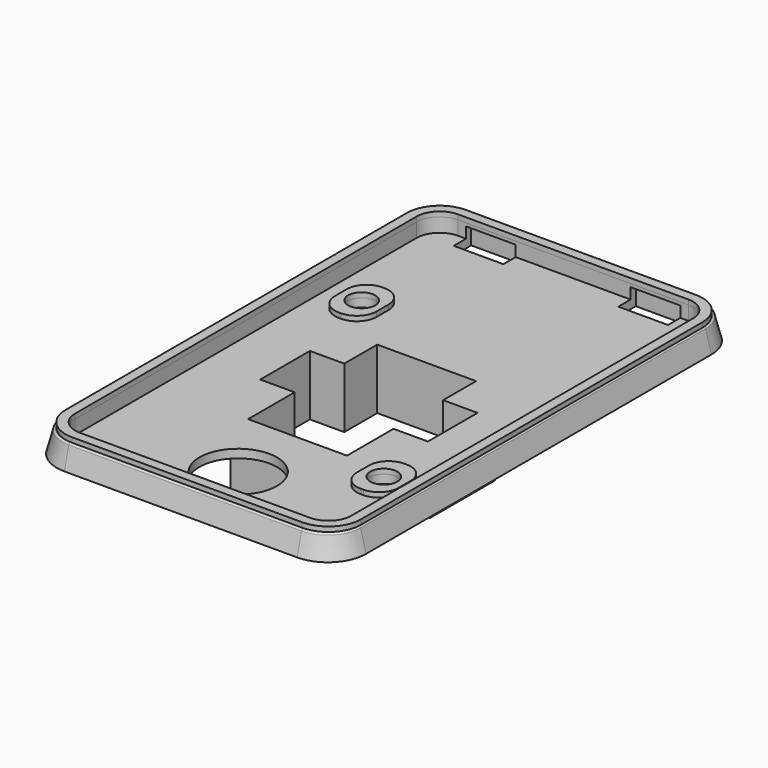
from build123d import *

# Parameters (mm, degrees)
F1_DEPTH     = 1
F4_DEPTH     = 4.64
F5_T1_DEPTH  = 48
F5_T3_DEPTH  = 89
F5_T6_ANGLE  = 90
F5_T8_ANGLE  = 90
F5_T10_ANGLE = 90
F5_T12_ANGLE = 90
F7_DEPTH     = 2.89
F8_R         = 0.4
F9_W         = 10.25
F9_H         = 4.5
F9_R         = 8
F9_R_2       = 2.8
F10_DEPTH    = 4
F11_R        = 2.7984324094
F11_R_2      = 2.7977753944
F12_DEPTH    = 1
F14_DEPTH    = 12.44
F16_DEPTH    = 1.75


# Not quite as in the source:
# - a fillet or chamfer that OpenCascade refuses, or shapes differently, is made with other operations: its cross-section is extruded or revolved along the edge and cut away or added


with BuildPart() as f1:
    # F0 (on Top) → F1 (new body)
    with BuildSketch(Plane.XY):
        with BuildLine():
            Line((23.75, 50.78), (0, 50.78))
            Line((0, 50.78), (-23.75, 50.78))
            ThreePointArc((-23.75, 50.78), (-28.522970773, 48.802970773), (-30.5, 44.03))
            Line((-30.5, 44.03), (-30.5, -44.03))
            ThreePointArc((-30.5, -44.03), (-28.522970773, -48.802970773), (-23.75, -50.78))
            Line((-23.75, -50.78), (0, -50.78))
            Line((0, -50.78), (23.75, -50.78))
            ThreePointArc((23.75, -50.78), (28.522970773, -48.802970773), (30.5, -44.03))
            Line((30.5, -44.03), (30.5, 44.03))
            ThreePointArc((30.5, 44.03), (28.522970773, 48.802970773), (23.75, 50.78))
        make_face()
        with BuildLine():
            Line((-23.75, 48.78), (0, 48.78))
            Line((0, 48.78), (23.75, 48.78))
            ThreePointArc((23.75, 48.78), (27.1087572106, 47.3887572106), (28.5, 44.03))
            Line((28.5, 44.03), (28.5, -44.03))
            ThreePointArc((28.5, -44.03), (27.1087572106, -47.3887572106), (23.75, -48.78))
            Line((23.75, -48.78), (0, -48.78))
            Line((0, -48.78), (-23.75, -48.78))
            ThreePointArc((-23.75, -48.78), (-27.1087572106, -47.3887572106), (-28.5, -44.03))
            Line((-28.5, -44.03), (-28.5, 44.03))
            ThreePointArc((-28.5, 44.03), (-27.1087572106, 47.3887572106), (-23.75, 48.78))
        make_face(mode=Mode.SUBTRACT)
    extrude(amount=F1_DEPTH)


with BuildPart() as f4:
    # F3 (on offset) → F4 (new body, through all)
    with BuildSketch(Plane(origin=(0, 0, -4.64), x_dir=(1, 0, 0), z_dir=(0, 0, -1))):
        with BuildLine():
            Line((24, 52.5), (0, 52.5))
            Line((0, 52.5), (-24, 52.5))
            ThreePointArc((-24, 52.5), (-29.6568542495, 50.1568542495), (-32, 44.5))
            Line((-32, 44.5), (-32, 0))
            Line((-32, 0), (-32, -44.5))
            ThreePointArc((-32, -44.5), (-29.6568542495, -50.1568542495), (-24, -52.5))
            Line((-24, -52.5), (0, -52.5))
            Line((0, -52.5), (24, -52.5))
            ThreePointArc((24, -52.5), (29.6568542495, -50.1568542495), (32, -44.5))
            Line((32, -44.5), (32, 0))
            Line((32, 0), (32, 44.5))
            ThreePointArc((32, 44.5), (29.6568542495, 50.1568542495), (24, 52.5))
        make_face()
    extrude(amount=-F4_DEPTH)

    # F5: chamfer of 1.3 x 5 on 8 edges, made by hand

    # F5_s2 → F5_t1 (cut)
    with BuildSketch(Plane.YZ.offset(-24)):
        Polygon((51.2, 0), (52.5, -5), (52.5, 0), align=None)
        Polygon((-51.2, 0), (-52.5, -5), (-52.5, 0), align=None)
    extrude(amount=F5_T1_DEPTH, mode=Mode.SUBTRACT)

    # F5_s4 → F5_t3 (cut)
    with BuildSketch(Plane.XZ.offset(-44.5)):
        Polygon((-30.7, 0), (-32, -5), (-32, 0), align=None)
        Polygon((30.7, 0), (32, -5), (32, 0), align=None)
    extrude(amount=F5_T3_DEPTH, mode=Mode.SUBTRACT)

    # F5_s5 → F5_t6 (revolve, cut)
    with BuildSketch(Plane.XZ.offset(44.5)):
        Polygon((32, -5), (30.7, 0), (32, 0), align=None)
    revolve(axis=Axis((24, -44.5, 0), (0, 0, -1)), revolution_arc=F5_T6_ANGLE, mode=Mode.SUBTRACT)

    # F5_s7 → F5_t8 (revolve, cut)
    with BuildSketch(Plane.YZ.offset(-24)):
        Polygon((-51.2, 0), (-52.5, -5), (-52.5, 0), align=None)
    revolve(axis=Axis((-24, -44.5, 0), (0, 0, -1)), revolution_arc=F5_T8_ANGLE, mode=Mode.SUBTRACT)

    # F5_s9 → F5_t10 (revolve, cut)
    with BuildSketch(Plane.XZ.offset(-44.5)):
        Polygon((-30.7, 0), (-32, -5), (-32, 0), align=None)
    revolve(axis=Axis((-24, 44.5, 0), (0, 0, -1)), revolution_arc=F5_T10_ANGLE, mode=Mode.SUBTRACT)

    # F5_s11 → F5_t12 (revolve, cut)
    with BuildSketch(Plane.YZ.offset(24)):
        Polygon((51.2, 0), (52.5, -5), (52.5, 0), align=None)
    revolve(axis=Axis((24, 44.5, 0), (0, 0, -1)), revolution_arc=F5_T12_ANGLE, mode=Mode.SUBTRACT)

    # F6 (on Top) → F7 (cut)
    with BuildSketch(Plane.XY):
        with BuildLine():
            Line((23.75, 48.78), (0, 48.78))
            Line((0, 48.78), (-23.75, 48.78))
            ThreePointArc((-23.75, 48.78), (-27.1087572106, 47.3887572106), (-28.5, 44.03))
            Line((-28.5, 44.03), (-28.5, -44.03))
            ThreePointArc((-28.5, -44.03), (-27.1087572106, -47.3887572106), (-23.75, -48.78))
            Line((-23.75, -48.78), (0, -48.78))
            Line((0, -48.78), (23.75, -48.78))
            ThreePointArc((23.75, -48.78), (27.1087572106, -47.3887572106), (28.5, -44.03))
            Line((28.5, -44.03), (28.5, 44.03))
            ThreePointArc((28.5, 44.03), (27.1087572106, 47.3887572106), (23.75, 48.78))
        make_face()
    extrude(amount=-F7_DEPTH, mode=Mode.SUBTRACT)

    # F8
    f8_edges = [f4.edges().sort_by_distance(p)[0] for p in [
        (0, -51.2, 0),
        (30.7, 0, 0),
        (28.737615, 49.237615, 0),
        (28.737615, -49.237615, 0),
        (0, 51.2, 0),
        (-28.737615, 49.237615, 0),
        (-30.7, 0, 0),
        (-28.737615, -49.237615, 0),
    ]]
    fillet(f8_edges, radius=F8_R)

    # F9 (on face) → F10 (cut)
    with BuildSketch(Plane(origin=(0, 0, -4.64), x_dir=(1, 0, 0), z_dir=(0, 0, -1))):
        with Locations((-16.9814, 47.8564)):
            Rectangle(F9_W, F9_H)
        with Locations((16.9814, 47.8564)):
            Rectangle(F9_W, F9_H)
        with Locations((-16.9814, -47.8564)):
            Rectangle(F9_W, F9_H)
        with Locations((16.9814, -47.8564)):
            Rectangle(F9_W, F9_H)
        with Locations((0, 37.5964)):
            Circle(F9_R)
        with Locations((20.6064, 25.8064)):
            Circle(F9_R_2)
        with Locations((-20.6064, -20.0064)):
            Circle(F9_R_2)
    extrude(amount=-F10_DEPTH, mode=Mode.SUBTRACT)

    # F11 (on face) → F12 (join)
    with BuildSketch(Plane.XY.offset(-2.89)):
        with BuildLine():
            Line((20.8564, -20.2064), (20.3564, -20.2064))
            ThreePointArc((20.3564, -20.2064), (17.4926175362, -21.3926175362), (16.3064, -24.2564))
            Line((16.3064, -24.2564), (16.3064, -27.3564))
            ThreePointArc((16.3064, -27.3564), (17.4926175362, -30.2201824638), (20.3564, -31.4064))
            Line((20.3564, -31.4064), (20.8564, -31.4064))
            ThreePointArc((20.8564, -31.4064), (23.7201824638, -30.2201824638), (24.9064, -27.3564))
            Line((24.9064, -27.3564), (24.9064, -24.2564))
            ThreePointArc((24.9064, -24.2564), (23.7201824638, -21.3926175362), (20.8564, -20.2064))
        make_face()
        with Locations((20.6064, -25.8064)):
            Circle(F11_R, mode=Mode.SUBTRACT)
        with BuildLine():
            Line((-20.3564, 25.6064), (-20.8564, 25.6064))
            ThreePointArc((-20.8564, 25.6064), (-23.7201824638, 24.4201824638), (-24.9064, 21.5564))
            Line((-24.9064, 21.5564), (-24.9064, 18.4564))
            ThreePointArc((-24.9064, 18.4564), (-23.7201824638, 15.5926175362), (-20.8564, 14.4064))
            Line((-20.8564, 14.4064), (-20.3564, 14.4064))
            ThreePointArc((-20.3564, 14.4064), (-17.4926175362, 15.5926175362), (-16.3064, 18.4564))
            Line((-16.3064, 18.4564), (-16.3064, 21.5564))
            ThreePointArc((-16.3064, 21.5564), (-17.4926175362, 24.4201824638), (-20.3564, 25.6064))
        make_face()
        with Locations((-20.6064, 20.0064)):
            Circle(F11_R_2, mode=Mode.SUBTRACT)
    extrude(amount=F12_DEPTH)

    # F13 (on face) → F14 (join)
    with BuildSketch(Plane.XY.offset(-2.89)):
        Polygon((12.2, 13.0036), (0, 13.0036), (-12.2, 13.0036), (-12.2, 4.5036), (-19.3, 4.5036), (-19.3, -12.2964), (-12.2, -12.2964), (-12.2, -24.2964), (0, -24.2964), (12.2, -24.2964), (12.2, -12.2964), (19.3, -12.2964), (19.3, 4.5036), (12.2, 4.5036), align=None)
        Polygon((10.2, -22.2964), (0, -22.2964), (-10.2, -22.2964), (-10.2, -10.2964), (-17.3, -10.2964), (-17.3, 2.5036), (-10.2, 2.5036), (-10.2, 11.0036), (0, 11.0036), (10.2, 11.0036), (10.2, 2.5036), (17.3, 2.5036), (17.3, -10.2964), (10.2, -10.2964), align=None, mode=Mode.SUBTRACT)
    extrude(amount=-F14_DEPTH)

    # F15 (on face) → F16 (cut, through all)
    with BuildSketch(Plane(origin=(0, 0, -4.64), x_dir=(1, 0, 0), z_dir=(0, 0, -1))):
        Polygon((10.2, 22.2964), (-10.2, 22.2964), (-10.2, 10.2964), (-17.3, 10.2964), (-17.3, -2.5036), (-10.2, -2.5036), (-10.2, -11.0036), (10.2, -11.0036), (10.2, -2.5036), (17.3, -2.5036), (17.3, 10.2964), (10.2, 10.2964), align=None)
    extrude(amount=-F16_DEPTH, mode=Mode.SUBTRACT)


solid = Compound([f1.part, f4.part])
